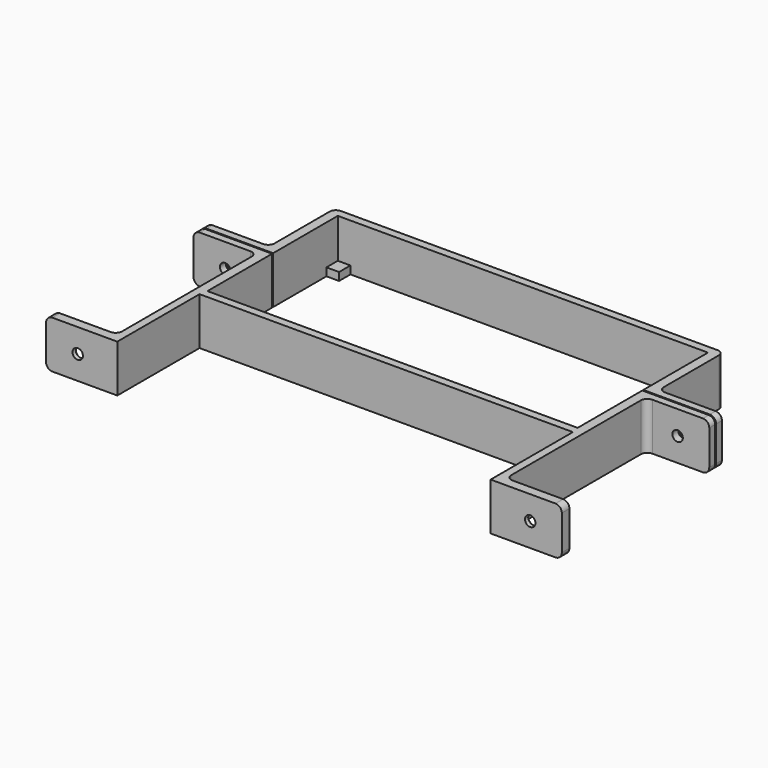
from build123d import *

# Parameters (mm, degrees)
F0_W            = 123
F0_H            = 56.5
F0_W_2          = 117
F0_H_2          = 51.5
F1_DEPTH        = 15
F3_W            = 2.5
F3_H            = 15
F4_DEPTH        = 32.5
F5_W            = 3
F5_H            = 15
F6_DEPTH        = 20
F7_W            = 3
F7_H            = 15
F8_DEPTH        = 20
F10_D           = 3.3
F10_DEPTH       = 5
F10_CSINK_D     = 6.72
F10_CSINK_ANGLE = 90
F10_TIP         = 0.9914200214
F12_D           = 3.3
F12_DEPTH       = 5
F12_CSINK_D     = 6.72
F12_CSINK_ANGLE = 90
F12_TIP         = 0.9914200214
F13_W           = 4
F13_H           = 4.5
F14_DEPTH       = 2.5
F15_W           = 5
F15_H           = 15
F16_DEPTH       = 20
F18_D           = 3.3
F18_CSINK_D     = 6.72
F18_CSINK_ANGLE = 90
F19_W           = 5
F19_H           = 15
F20_DEPTH       = 20
F22_D           = 3.3
F22_CSINK_D     = 6.72
F22_CSINK_ANGLE = 90
F23_W           = 0.4
F23_H           = 15
F24_DEPTH       = 200
F25_R           = 2


with BuildPart() as f1:
    # F0 (on Top) → F1 (new body)
    with BuildSketch(Plane.XY):
        Rectangle(F0_W, F0_H)
        Rectangle(F0_W_2, F0_H_2, mode=Mode.SUBTRACT)
    extrude(amount=F1_DEPTH)

    # F3 (on face) → F4 (join)
    with BuildSketch(Plane.XZ.offset(28.25)):
        with Locations((-60.25, 7.5)):
            Rectangle(F3_W, F3_H)
        with Locations((60.25, 7.5)):
            Rectangle(F3_W, F3_H)
    extrude(amount=F4_DEPTH)

    # F5 (on face) → F6 (join)
    with BuildSketch(Plane(origin=(-61.5, 0, 0), x_dir=(0, -1, 0), z_dir=(-1, 0, 0))):
        with Locations((59.25, 7.5)):
            Rectangle(F5_W, F5_H)
    extrude(amount=F6_DEPTH)

    # F7 (on face) → F8 (join)
    with BuildSketch(Plane.YZ.offset(61.5)):
        with Locations((-59.25, 7.5)):
            Rectangle(F7_W, F7_H)
    extrude(amount=F8_DEPTH)

    # F10
    with Locations(Plane(origin=(0, -57.75, 0), x_dir=(-1, 0, 0), z_dir=(0, 1, 0))):
        with Locations((-71.5, 7.5)):
            CounterSinkHole(F10_D / 2, F10_CSINK_D / 2, depth=F10_DEPTH, counter_sink_angle=F10_CSINK_ANGLE)
            with Locations((0, 0, -(F10_DEPTH + F10_TIP / 2))):  # 118° drill point
                Cone(0, F10_D / 2, F10_TIP, mode=Mode.SUBTRACT)

    # F12
    with Locations(Plane(origin=(0, -57.75, 0), x_dir=(-1, 0, 0), z_dir=(0, 1, 0))):
        with Locations((71.5, 7.5)):
            CounterSinkHole(F12_D / 2, F12_CSINK_D / 2, depth=F12_DEPTH, counter_sink_angle=F12_CSINK_ANGLE)
            with Locations((0, 0, -(F12_DEPTH + F12_TIP / 2))):  # 118° drill point
                Cone(0, F12_D / 2, F12_TIP, mode=Mode.SUBTRACT)

    # F13 (on face) → F14 (join)
    with BuildSketch(Plane(origin=(0, 0, 0), x_dir=(1, 0, 0), z_dir=(0, 0, -1))):
        with Locations((-56.5, -23.5)):
            Rectangle(F13_W, F13_H)
        with Locations((-56.5, 23.5)):
            Rectangle(F13_W, F13_H)
        with Locations((56.5, 23.5)):
            Rectangle(F13_W, F13_H)
        with Locations((56.5, -23.5)):
            Rectangle(F13_W, F13_H)
    extrude(amount=-F14_DEPTH)

    # F15 (on face) → F16 (join)
    with BuildSketch(Plane(origin=(-61.5, 0, 0), x_dir=(0, -1, 0), z_dir=(-1, 0, 0))):
        with Locations((0, 7.5)):
            Rectangle(F15_W, F15_H)
    extrude(amount=F16_DEPTH)

    # F18 (through all)
    with Locations(Plane(origin=(0, 2.5, 0), x_dir=(-1, 0, 0), z_dir=(0, 1, 0))):
        with Locations((71.5, 7.5)):
            CounterSinkHole(F18_D / 2, F18_CSINK_D / 2, counter_sink_angle=F18_CSINK_ANGLE)

    # F19 (on face) → F20 (join)
    with BuildSketch(Plane.YZ.offset(61.5)):
        with Locations((0, 7.5)):
            Rectangle(F19_W, F19_H)
    extrude(amount=F20_DEPTH)

    # F22 (through all)
    with Locations(Plane(origin=(0, 2.5, 0), x_dir=(-1, 0, 0), z_dir=(0, 1, 0))):
        with Locations((-71.5, 7.5)):
            CounterSinkHole(F22_D / 2, F22_CSINK_D / 2, counter_sink_angle=F22_CSINK_ANGLE)

    # F23 (on face) → F24 (cut)
    with BuildSketch(Plane.YZ.offset(81.5)):
        with Locations((0, 7.5)):
            Rectangle(F23_W, F23_H)
    extrude(amount=-F24_DEPTH, mode=Mode.SUBTRACT)

    # F25
    f25_edges = [f1.edges().sort_by_distance(p)[0] for p in [
        (-61.5, 28.25, 7.5),
        (-81.5, -1.35, 0),
        (-81.5, 1.35, 0),
        (-81.5, -59.25, 15),
        (81.5, -59.25, 0),
        (81.5, -1.35, 15),
        (81.5, 1.35, 15),
        (61.5, 28.25, 7.5),
        (-61.5, -57.75, 7.5),
        (61.5, -57.75, 7.5),
        (81.5, -1.35, 0),
        (81.5, 1.35, 0),
        (-81.5, -1.35, 15),
        (-81.5, 1.35, 15),
        (-61.5, 2.5, 7.5),
        (-61.5, -2.5, 7.5),
        (61.5, 2.5, 7.5),
        (61.5, -2.5, 7.5),
        (-81.5, -59.25, 0),
        (81.5, -59.25, 15),
    ]]
    fillet(f25_edges, radius=F25_R)


solid = f1.part
